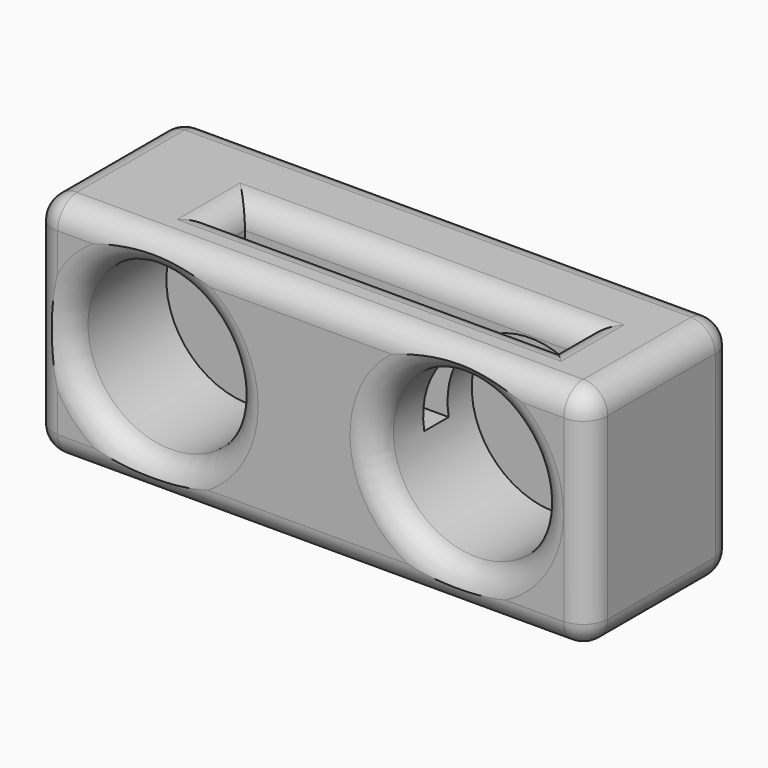
from build123d import *

# Parameters (mm, degrees)
F0_W          = 134.4953402877
F0_H          = 47.3678857088
F1_DEPTH      = 38.1
F2_R          = 17.202838431
F3_DEPTH      = 25.4
F4_W          = 69.85
F4_H          = 6.35
F5_DEPTH      = 25.4
F6_DEPTH      = 19.05
F7_T1_DEPTH   = 105.2834089168
F7_T3_DEPTH   = 27.9380686292
F7_T5_DEPTH   = 37.205954338
F7_T7_DEPTH   = 69.85
F7_T9_DEPTH   = 6.35
F7_S13_W      = 5.589502254
F7_S13_H      = 5.5895022539
F7_T14_DEPTH  = 5.589502254
F7_S19_W      = 5.5895022539
F7_S19_H      = 5.589502254
F7_T20_DEPTH  = 5.589502254
F7_S25_W      = 5.589502254
F7_S25_H      = 5.5895022539
F7_T26_DEPTH  = 5.589502254
F7_S31_W      = 5.5895022539
F7_S31_H      = 5.589502254
F7_T32_DEPTH  = 5.589502254
F7_S37_W      = 5.589502254
F7_S37_H      = 5.5895022539
F7_T38_DEPTH  = 5.589502254
F7_S43_W      = 5.5895022539
F7_S43_H      = 5.5895022539
F7_T44_DEPTH  = 5.589502254
F7_S49_W      = 5.589502254
F7_S49_H      = 5.5895022539
F7_T50_DEPTH  = 5.589502254
F7_S55_W      = 5.5895022539
F7_S55_H      = 5.5895022539
F7_T56_DEPTH  = 5.589502254
F7_T67_DEPTH  = 82.5524142529
F7_T71_DEPTH  = 19.0524142529
F7_T78_DEPTH  = 82.5524142529
F7_T82_DEPTH  = 19.0524142529
F7_T89_DEPTH  = 19.0524142529
F7_T93_DEPTH  = 82.5524142529
F7_T100_DEPTH = 19.0524142529
F7_T104_DEPTH = 82.5524142529


# Not quite as in the source:
# - a fillet or chamfer that OpenCascade refuses, or shapes differently, is made with other operations: its cross-section is extruded or revolved along the edge and cut away or added


with BuildPart() as f1:
    # F0 (on Front) → F1 (new body)
    with BuildSketch(Plane.XZ):
        with Locations((1.4725737274, 23.6839428544)):
            Rectangle(F0_W, F0_H)
    extrude(amount=F1_DEPTH)

    # F2 (on face) → F3 (cut)
    with BuildSketch(Plane.XZ.offset(38.1)):
        with Locations((-41.2180274725, 23.8331388682)):
            Circle(F2_R)
        with Locations((22.3340820521, 24.7883740813)):
            Circle(F2_R)
    extrude(amount=-F3_DEPTH, mode=Mode.SUBTRACT)

    # F4 (on face) → F5 (cut)
    with BuildSketch(Plane.XY.offset(47.3678857088)):
        with Locations((-2.1010648489, -22.1751800656)):
            Rectangle(F4_W, F4_H)
    extrude(amount=-F5_DEPTH, mode=Mode.SUBTRACT)

    # F6 (cut): a face of the model
    f6_faces = [f1.faces().sort_by_distance(p)[0] for p in [
        (68.7202438712, -19.05, 23.6839428544),
    ]]
    extrude(f6_faces, amount=-F6_DEPTH, mode=Mode.SUBTRACT)

    # F7: fillet of radius 5.08 on 18 edges, made by hand

    # F7_s2 → F7_t1 (cut)
    with BuildSketch(Plane.YZ.offset(-60.694130731)):
        with BuildLine():
            ThreePointArc((-33.0190343146, 47.3682857088), (-36.6121024484, 45.8799881572), (-38.1004, 42.2869200234))
            Line((-38.1004, 42.2869200234), (-38.6085365685, 42.2869200234))
            ThreePointArc((-38.6085365685, 42.2869200234), (-38.6081365685, 44.8274028661), (-38.6081365685, 47.3678857088))
            Line((-38.6081365685, 47.3678857088), (-38.1, 47.8760222774))
            ThreePointArc((-38.1, 47.8760222774), (-35.5595171573, 47.8760222774), (-33.0190343146, 47.8764222774))
            Line((-33.0190343146, 47.8764222774), (-33.0190343146, 47.3682857088))
        make_face()
        with BuildLine():
            ThreePointArc((-5.0809656854, 47.3682857088), (-1.4878975516, 45.8799881572), (0.0004, 42.2869200234))
            Line((0.0004, 42.2869200234), (0.5085365685, 42.2869200234))
            ThreePointArc((0.5085365685, 42.2869200234), (0.5081365685, 44.8274028661), (0.5081365685, 47.3678857088))
            Line((0.5081365685, 47.3678857088), (0, 47.8760222774))
            ThreePointArc((0, 47.8760222774), (-2.5404828427, 47.8760222774), (-5.0809656854, 47.8764222774))
            Line((-5.0809656854, 47.8764222774), (-5.0809656854, 47.3682857088))
        make_face()
        with BuildLine():
            ThreePointArc((-33.0190343146, -0.0004), (-36.6121024484, 1.4878975516), (-38.1004, 5.0809656854))
            Line((-38.1004, 5.0809656854), (-38.6085365685, 5.0809656854))
            ThreePointArc((-38.6085365685, 5.0809656854), (-38.6081365685, 2.5404828427), (-38.6081365685, 0))
            Line((-38.6081365685, 0), (-38.1, -0.5081365685))
            ThreePointArc((-38.1, -0.5081365685), (-35.5595171573, -0.5081365685), (-33.0190343146, -0.5085365685))
            Line((-33.0190343146, -0.5085365685), (-33.0190343146, -0.0004))
        make_face()
        with BuildLine():
            ThreePointArc((-5.0809656854, -0.0004), (-1.4878975516, 1.4878975516), (0.0004, 5.0809656854))
            Line((0.0004, 5.0809656854), (0.5085365685, 5.0809656854))
            ThreePointArc((0.5085365685, 5.0809656854), (0.5081365685, 2.5404828427), (0.5081365685, 0))
            Line((0.5081365685, 0), (0, -0.5081365685))
            ThreePointArc((0, -0.5081365685), (-2.5404828427, -0.5081365685), (-5.0809656854, -0.5085365685))
            Line((-5.0809656854, -0.5085365685), (-5.0809656854, -0.0004))
        make_face()
    extrude(amount=F7_T1_DEPTH, mode=Mode.SUBTRACT)

    # F7_s4 → F7_t3 (cut)
    with BuildSketch(Plane.XZ.offset(5.0809656854)):
        with BuildLine():
            ThreePointArc((44.5892781858, 47.3682857088), (48.1823463196, 45.8799881572), (49.6706438712, 42.2869200234))
            Line((49.6706438712, 42.2869200234), (50.1787804398, 42.2869200234))
            ThreePointArc((50.1787804398, 42.2869200234), (50.1783804398, 44.8274028661), (50.1783804398, 47.3678857088))
            Line((50.1783804398, 47.3678857088), (49.6702438712, 47.8760222774))
            ThreePointArc((49.6702438712, 47.8760222774), (47.1297610285, 47.8760222774), (44.5892781858, 47.8764222774))
            Line((44.5892781858, 47.8764222774), (44.5892781858, 47.3682857088))
        make_face()
        with BuildLine():
            ThreePointArc((-65.7754964165, 42.2869200234), (-64.2871988649, 45.8799881572), (-60.694130731, 47.3682857088))
            Line((-60.694130731, 47.3682857088), (-60.694130731, 47.8764222774))
            ThreePointArc((-60.694130731, 47.8764222774), (-63.2346135738, 47.8760222774), (-65.7750964165, 47.8760222774))
            Line((-65.7750964165, 47.8760222774), (-66.283232985, 47.3678857088))
            ThreePointArc((-66.283232985, 47.3678857088), (-66.283232985, 44.8274028661), (-66.283632985, 42.2869200234))
            Line((-66.283632985, 42.2869200234), (-65.7754964165, 42.2869200234))
        make_face()
        with BuildLine():
            ThreePointArc((44.5892781858, -0.0004), (48.1823463196, 1.4878975516), (49.6706438712, 5.0809656854))
            Line((49.6706438712, 5.0809656854), (50.1787804398, 5.0809656854))
            ThreePointArc((50.1787804398, 5.0809656854), (50.1783804398, 2.5404828427), (50.1783804398, 0))
            Line((50.1783804398, 0), (49.6702438712, -0.5081365685))
            ThreePointArc((49.6702438712, -0.5081365685), (47.1297610285, -0.5081365685), (44.5892781858, -0.5085365685))
            Line((44.5892781858, -0.5085365685), (44.5892781858, -0.0004))
        make_face()
        with BuildLine():
            ThreePointArc((-65.7754964165, 5.0809656854), (-64.2871988649, 1.4878975516), (-60.694130731, -0.0004))
            Line((-60.694130731, -0.0004), (-60.694130731, -0.5085365685))
            ThreePointArc((-60.694130731, -0.5085365685), (-63.2346135738, -0.5081365685), (-65.7750964165, -0.5081365685))
            Line((-65.7750964165, -0.5081365685), (-66.283232985, 0))
            ThreePointArc((-66.283232985, 0), (-66.283232985, 2.5404828427), (-66.283632985, 5.0809656854))
            Line((-66.283632985, 5.0809656854), (-65.7754964165, 5.0809656854))
        make_face()
    extrude(amount=F7_T3_DEPTH, mode=Mode.SUBTRACT)

    # F7_s6 → F7_t5 (cut)
    with BuildSketch(Plane.XY.offset(5.0809656854)):
        with BuildLine():
            ThreePointArc((44.5892781858, -38.1004), (48.1823463196, -36.6121024484), (49.6706438712, -33.0190343146))
            Line((49.6706438712, -33.0190343146), (50.1787804398, -33.0190343146))
            ThreePointArc((50.1787804398, -33.0190343146), (50.1783804398, -35.5595171573), (50.1783804398, -38.1))
            Line((50.1783804398, -38.1), (49.6702438712, -38.6081365685))
            ThreePointArc((49.6702438712, -38.6081365685), (47.1297610285, -38.6081365685), (44.5892781858, -38.6085365685))
            Line((44.5892781858, -38.6085365685), (44.5892781858, -38.1004))
        make_face()
        with BuildLine():
            ThreePointArc((-65.7754964165, -33.0190343146), (-64.2871988649, -36.6121024484), (-60.694130731, -38.1004))
            Line((-60.694130731, -38.1004), (-60.694130731, -38.6085365685))
            ThreePointArc((-60.694130731, -38.6085365685), (-63.2346135738, -38.6081365685), (-65.7750964165, -38.6081365685))
            Line((-65.7750964165, -38.6081365685), (-66.283232985, -38.1))
            ThreePointArc((-66.283232985, -38.1), (-66.283232985, -35.5595171573), (-66.283632985, -33.0190343146))
            Line((-66.283632985, -33.0190343146), (-65.7754964165, -33.0190343146))
        make_face()
        with BuildLine():
            ThreePointArc((44.5892781858, 0.0004), (48.1823463196, -1.4878975516), (49.6706438712, -5.0809656854))
            Line((49.6706438712, -5.0809656854), (50.1787804398, -5.0809656854))
            ThreePointArc((50.1787804398, -5.0809656854), (50.1783804398, -2.5404828427), (50.1783804398, 0))
            Line((50.1783804398, 0), (49.6702438712, 0.5081365685))
            ThreePointArc((49.6702438712, 0.5081365685), (47.1297610285, 0.5081365685), (44.5892781858, 0.5085365685))
            Line((44.5892781858, 0.5085365685), (44.5892781858, 0.0004))
        make_face()
        with BuildLine():
            ThreePointArc((-65.7754964165, -5.0809656854), (-64.2871988649, -1.4878975516), (-60.694130731, 0.0004))
            Line((-60.694130731, 0.0004), (-60.694130731, 0.5085365685))
            ThreePointArc((-60.694130731, 0.5085365685), (-63.2346135738, 0.5081365685), (-65.7750964165, 0.5081365685))
            Line((-65.7750964165, 0.5081365685), (-66.283232985, 0))
            ThreePointArc((-66.283232985, 0), (-66.283232985, -2.5404828427), (-66.283632985, -5.0809656854))
            Line((-66.283632985, -5.0809656854), (-65.7754964165, -5.0809656854))
        make_face()
    extrude(amount=F7_T5_DEPTH, mode=Mode.SUBTRACT)

    # F7_s8 → F7_t7 (cut)
    with BuildSketch(Plane.YZ.offset(-37.0260648489)):
        with BuildLine():
            ThreePointArc((-30.4311457511, 47.3682857088), (-26.8380776172, 45.8799881572), (-25.3497800656, 42.2869200234))
            Line((-25.3497800656, 42.2869200234), (-24.8416434971, 42.2869200234))
            ThreePointArc((-24.8416434971, 42.2869200234), (-24.8420434971, 44.8274028661), (-24.8420434971, 47.3678857088))
            Line((-24.8420434971, 47.3678857088), (-25.3501800656, 47.8760222774))
            ThreePointArc((-25.3501800656, 47.8760222774), (-27.8906629083, 47.8760222774), (-30.4311457511, 47.8764222774))
            Line((-30.4311457511, 47.8764222774), (-30.4311457511, 47.3682857088))
        make_face()
        with BuildLine():
            ThreePointArc((-13.9192143802, 47.3682857088), (-17.5122825141, 45.8799881572), (-19.0005800656, 42.2869200234))
            Line((-19.0005800656, 42.2869200234), (-19.5087166342, 42.2869200234))
            ThreePointArc((-19.5087166342, 42.2869200234), (-19.5083166342, 44.8274028661), (-19.5083166342, 47.3678857088))
            Line((-19.5083166342, 47.3678857088), (-19.0001800656, 47.8760222774))
            ThreePointArc((-19.0001800656, 47.8760222774), (-16.4596972229, 47.8760222774), (-13.9192143802, 47.8764222774))
            Line((-13.9192143802, 47.8764222774), (-13.9192143802, 47.3682857088))
        make_face()
    extrude(amount=F7_T7_DEPTH, mode=Mode.SUBTRACT)

    # F7_s10 → F7_t9 (cut)
    with BuildSketch(Plane.XZ.offset(19.0001800656)):
        with BuildLine():
            ThreePointArc((37.9049008365, 47.3682857088), (34.3118327027, 45.8799881572), (32.8235351511, 42.2869200234))
            Line((32.8235351511, 42.2869200234), (32.3153985826, 42.2869200234))
            ThreePointArc((32.3153985826, 42.2869200234), (32.3157985826, 44.8274028661), (32.3157985826, 47.3678857088))
            Line((32.3157985826, 47.3678857088), (32.8239351511, 47.8760222774))
            ThreePointArc((32.8239351511, 47.8760222774), (35.3644179938, 47.8760222774), (37.9049008365, 47.8764222774))
            Line((37.9049008365, 47.8764222774), (37.9049008365, 47.3682857088))
        make_face()
        with BuildLine():
            ThreePointArc((-42.1070305343, 47.3682857088), (-38.5139624005, 45.8799881572), (-37.0256648489, 42.2869200234))
            Line((-37.0256648489, 42.2869200234), (-36.5175282804, 42.2869200234))
            ThreePointArc((-36.5175282804, 42.2869200234), (-36.5179282804, 44.8274028661), (-36.5179282804, 47.3678857088))
            Line((-36.5179282804, 47.3678857088), (-37.0260648489, 47.8760222774))
            ThreePointArc((-37.0260648489, 47.8760222774), (-39.5665476916, 47.8760222774), (-42.1070305343, 47.8764222774))
            Line((-42.1070305343, 47.8764222774), (-42.1070305343, 47.3682857088))
        make_face()
    extrude(amount=F7_T9_DEPTH, mode=Mode.SUBTRACT)


with BuildPart() as f7_tool12:
    # F7_s13 → F7_t14 (new body)
    with BuildSketch(Plane.XY.offset(42.2869200234)):
        with Locations((47.3840293128, -35.8137854415)):
            Rectangle(F7_S13_W, F7_S13_H)
    extrude(amount=F7_T14_DEPTH)

    # F7_s15 → F7_t16 (revolve, cut)
    with BuildSketch(Plane(origin=(44.5892781858, -33.0190343146, 42.2869200234), x_dir=(-0.7071067812, 0.7071067812, 0), z_dir=(0.7071067812, 0.7071067812, 0))):
        with BuildLine():
            ThreePointArc((0, -5.0813656854), (5.0813656854, 0), (0, 5.0813656854))
            Line((0, 5.0813656854), (0, -5.0813656854))
        make_face()
    revolve(axis=Axis((44.5892781858, -33.0190343146, 42.2869200234), (0, 0, 1)), mode=Mode.SUBTRACT)


with BuildPart() as f1_1:
    add(f1.part)

    # F7_t11: cut F7_tool12
    add(f7_tool12.part, mode=Mode.SUBTRACT)


with BuildPart() as f7_tool18:
    # F7_s19 → F7_t20 (new body)
    with BuildSketch(Plane.YZ.offset(-60.694130731)):
        with Locations((-35.8137854415, 45.0816711504)):
            Rectangle(F7_S19_W, F7_S19_H)
    extrude(amount=-F7_T20_DEPTH)

    # F7_s21 → F7_t22 (revolve, cut)
    with BuildSketch(Plane(origin=(-60.694130731, -33.0190343146, 42.2869200234), x_dir=(0, 0.7071067812, -0.7071067812), z_dir=(0, 0.7071067812, 0.7071067812))):
        with BuildLine():
            ThreePointArc((0, -5.0813656854), (5.0813656854, 0), (0, 5.0813656854))
            Line((0, 5.0813656854), (0, -5.0813656854))
        make_face()
    revolve(axis=Axis((-60.694130731, -33.0190343146, 42.2869200234), (-1, 0, 0)), mode=Mode.SUBTRACT)


with BuildPart() as f1_2:
    add(f1_1.part)

    # F7_t17: cut F7_tool18
    add(f7_tool18.part, mode=Mode.SUBTRACT)


with BuildPart() as f7_tool24:
    # F7_s25 → F7_t26 (new body)
    with BuildSketch(Plane.XY.offset(42.2869200234)):
        with Locations((47.3840293128, -2.2862145584)):
            Rectangle(F7_S25_W, F7_S25_H)
    extrude(amount=F7_T26_DEPTH)

    # F7_s27 → F7_t28 (revolve, cut)
    with BuildSketch(Plane(origin=(44.5892781858, -5.0809656854, 42.2869200234), x_dir=(-0.7071067812, -0.7071067812, 0), z_dir=(-0.7071067812, 0.7071067812, 0))):
        with BuildLine():
            ThreePointArc((0, -5.0813656854), (5.0813656854, 0), (0, 5.0813656854))
            Line((0, 5.0813656854), (0, -5.0813656854))
        make_face()
    revolve(axis=Axis((44.5892781858, -5.0809656854, 42.2869200234), (0, 0, 1)), mode=Mode.SUBTRACT)


with BuildPart() as f1_3:
    add(f1_2.part)

    # F7_t23: cut F7_tool24
    add(f7_tool24.part, mode=Mode.SUBTRACT)


with BuildPart() as f7_tool30:
    # F7_s31 → F7_t32 (new body)
    with BuildSketch(Plane.YZ.offset(-60.694130731)):
        with Locations((-2.2862145584, 45.0816711504)):
            Rectangle(F7_S31_W, F7_S31_H)
    extrude(amount=-F7_T32_DEPTH)

    # F7_s33 → F7_t34 (revolve, cut)
    with BuildSketch(Plane(origin=(-60.694130731, -5.0809656854, 42.2869200234), x_dir=(0, -0.7071067812, -0.7071067812), z_dir=(0, 0.7071067812, -0.7071067812))):
        with BuildLine():
            ThreePointArc((0, -5.0813656854), (5.0813656854, 0), (0, 5.0813656854))
            Line((0, 5.0813656854), (0, -5.0813656854))
        make_face()
    revolve(axis=Axis((-60.694130731, -5.0809656854, 42.2869200234), (-1, 0, 0)), mode=Mode.SUBTRACT)


with BuildPart() as f1_4:
    add(f1_3.part)

    # F7_t29: cut F7_tool30
    add(f7_tool30.part, mode=Mode.SUBTRACT)


with BuildPart() as f7_tool36:
    # F7_s37 → F7_t38 (new body)
    with BuildSketch(Plane.XY.offset(5.0809656854)):
        with Locations((47.3840293128, -35.8137854415)):
            Rectangle(F7_S37_W, F7_S37_H)
    extrude(amount=-F7_T38_DEPTH)

    # F7_s39 → F7_t40 (revolve, cut)
    with BuildSketch(Plane(origin=(44.5892781858, -33.0190343146, 5.0809656854), x_dir=(-0.7071067812, 0.7071067812, 0), z_dir=(-0.7071067812, -0.7071067812, 0))):
        with BuildLine():
            ThreePointArc((0, -5.0813656854), (5.0813656854, 0), (0, 5.0813656854))
            Line((0, 5.0813656854), (0, -5.0813656854))
        make_face()
    revolve(axis=Axis((44.5892781858, -33.0190343146, 5.0809656854), (0, 0, -1)), mode=Mode.SUBTRACT)


with BuildPart() as f1_5:
    add(f1_4.part)

    # F7_t35: cut F7_tool36
    add(f7_tool36.part, mode=Mode.SUBTRACT)


with BuildPart() as f7_tool42:
    # F7_s43 → F7_t44 (new body)
    with BuildSketch(Plane.YZ.offset(-60.694130731)):
        with Locations((-35.8137854415, 2.2862145584)):
            Rectangle(F7_S43_W, F7_S43_H)
    extrude(amount=-F7_T44_DEPTH)

    # F7_s45 → F7_t46 (revolve, cut)
    with BuildSketch(Plane(origin=(-60.694130731, -33.0190343146, 5.0809656854), x_dir=(0, 0.7071067812, 0.7071067812), z_dir=(0, -0.7071067812, 0.7071067812))):
        with BuildLine():
            ThreePointArc((0, -5.0813656854), (5.0813656854, 0), (0, 5.0813656854))
            Line((0, 5.0813656854), (0, -5.0813656854))
        make_face()
    revolve(axis=Axis((-60.694130731, -33.0190343146, 5.0809656854), (-1, 0, 0)), mode=Mode.SUBTRACT)


with BuildPart() as f1_6:
    add(f1_5.part)

    # F7_t41: cut F7_tool42
    add(f7_tool42.part, mode=Mode.SUBTRACT)


with BuildPart() as f7_tool48:
    # F7_s49 → F7_t50 (new body)
    with BuildSketch(Plane.XY.offset(5.0809656854)):
        with Locations((47.3840293128, -2.2862145584)):
            Rectangle(F7_S49_W, F7_S49_H)
    extrude(amount=-F7_T50_DEPTH)

    # F7_s51 → F7_t52 (revolve, cut)
    with BuildSketch(Plane(origin=(44.5892781858, -5.0809656854, 5.0809656854), x_dir=(-0.7071067812, -0.7071067812, 0), z_dir=(0.7071067812, -0.7071067812, 0))):
        with BuildLine():
            ThreePointArc((0, -5.0813656854), (5.0813656854, 0), (0, 5.0813656854))
            Line((0, 5.0813656854), (0, -5.0813656854))
        make_face()
    revolve(axis=Axis((44.5892781858, -5.0809656854, 5.0809656854), (0, 0, -1)), mode=Mode.SUBTRACT)


with BuildPart() as f1_7:
    add(f1_6.part)

    # F7_t47: cut F7_tool48
    add(f7_tool48.part, mode=Mode.SUBTRACT)


with BuildPart() as f7_tool54:
    # F7_s55 → F7_t56 (new body)
    with BuildSketch(Plane.YZ.offset(-60.694130731)):
        with Locations((-2.2862145584, 2.2862145584)):
            Rectangle(F7_S55_W, F7_S55_H)
    extrude(amount=-F7_T56_DEPTH)

    # F7_s57 → F7_t58 (revolve, cut)
    with BuildSketch(Plane(origin=(-60.694130731, -5.0809656854, 5.0809656854), x_dir=(0, -0.7071067812, 0.7071067812), z_dir=(0, -0.7071067812, -0.7071067812))):
        with BuildLine():
            ThreePointArc((0, -5.0813656854), (5.0813656854, 0), (0, 5.0813656854))
            Line((0, 5.0813656854), (0, -5.0813656854))
        make_face()
    revolve(axis=Axis((-60.694130731, -5.0809656854, 5.0809656854), (-1, 0, 0)), mode=Mode.SUBTRACT)


with BuildPart() as f1_8:
    add(f1_7.part)

    # F7_t53: cut F7_tool54
    add(f7_tool54.part, mode=Mode.SUBTRACT)

    # F7_s59 → F7_t60 (revolve, cut)
    with BuildSketch(Plane.XY.offset(23.8331388682)):
        with BuildLine():
            ThreePointArc((-18.9342233561, -38.1004), (-22.52729149, -36.6121024484), (-24.0155890415, -33.0190343146))
            Line((-24.0155890415, -33.0190343146), (-24.5237256101, -33.0190343146))
            ThreePointArc((-24.5237256101, -33.0190343146), (-24.5233256101, -35.5595171573), (-24.5233256101, -38.1))
            Line((-24.5233256101, -38.1), (-24.0151890415, -38.6081365685))
            ThreePointArc((-24.0151890415, -38.6081365685), (-21.4747061988, -38.6081365685), (-18.9342233561, -38.6085365685))
            Line((-18.9342233561, -38.6085365685), (-18.9342233561, -38.1004))
        make_face()
    revolve(axis=Axis((-41.2180274725, -38.1, 23.8331388682), (0, -1, 0)), mode=Mode.SUBTRACT)

    # F7_s61 → F7_t62 (revolve, cut)
    with BuildSketch(Plane.XY.offset(24.7883740813)):
        with BuildLine():
            ThreePointArc((44.6178861685, -38.1004), (41.0248180346, -36.6121024484), (39.5365204831, -33.0190343146))
            Line((39.5365204831, -33.0190343146), (39.0283839145, -33.0190343146))
            ThreePointArc((39.0283839145, -33.0190343146), (39.0287839145, -35.5595171573), (39.0287839145, -38.1))
            Line((39.0287839145, -38.1), (39.5369204831, -38.6081365685))
            ThreePointArc((39.5369204831, -38.6081365685), (42.0774033258, -38.6081365685), (44.6178861685, -38.6085365685))
            Line((44.6178861685, -38.6085365685), (44.6178861685, -38.1004))
        make_face()
    revolve(axis=Axis((22.3340820521, -38.1, 24.7883740813), (0, -1, 0)), mode=Mode.SUBTRACT)


with BuildPart() as f7_tool65:
    # F7_s66 → F7_t67 (new body)
    with BuildSketch(Plane.YZ.offset(-49.7284791018)):
        with BuildLine():
            ThreePointArc((-30.4311457511, 47.3682857088), (-26.8380776172, 45.8799881572), (-25.3497800656, 42.2869200234))
            Line((-25.3497800656, 42.2869200234), (-24.8416434971, 42.2869200234))
            ThreePointArc((-24.8416434971, 42.2869200234), (-24.8420434971, 44.8274028661), (-24.8420434971, 47.3678857088))
            Line((-24.8420434971, 47.3678857088), (-25.3501800656, 47.8760222774))
            ThreePointArc((-25.3501800656, 47.8760222774), (-27.8906629083, 47.8760222774), (-30.4311457511, 47.8764222774))
            Line((-30.4311457511, 47.8764222774), (-30.4311457511, 47.3682857088))
        make_face()
    extrude(amount=F7_T67_DEPTH)

    split(bisect_by=Plane.YZ.offset(-37.0260648489), keep=Keep.BOTTOM)


with BuildPart() as f7_tool69:
    # F7_s70 → F7_t71 (new body)
    with BuildSketch(Plane.XZ.offset(19.0001800656)):
        with BuildLine():
            ThreePointArc((-42.1070305343, 47.3682857088), (-38.5139624005, 45.8799881572), (-37.0256648489, 42.2869200234))
            Line((-37.0256648489, 42.2869200234), (-36.5175282804, 42.2869200234))
            ThreePointArc((-36.5175282804, 42.2869200234), (-36.5179282804, 44.8274028661), (-36.5179282804, 47.3678857088))
            Line((-36.5179282804, 47.3678857088), (-37.0260648489, 47.8760222774))
            ThreePointArc((-37.0260648489, 47.8760222774), (-39.5665476916, 47.8760222774), (-42.1070305343, 47.8764222774))
            Line((-42.1070305343, 47.8764222774), (-42.1070305343, 47.3682857088))
        make_face()
    extrude(amount=F7_T71_DEPTH)

    split(bisect_by=Plane.XZ.offset(25.3501800656), keep=Keep.TOP)


with BuildPart() as f7_tool65_1:
    add(f7_tool65.part)

    # F7_t73: intersect F7_tool69
    add(f7_tool69.part, mode=Mode.INTERSECT)


with BuildPart() as f1_9:
    add(f1_8.part)

    # F7_t63: cut F7_tool65
    add(f7_tool65_1.part, mode=Mode.SUBTRACT)


with BuildPart() as f7_tool76:
    # F7_s77 → F7_t78 (new body)
    with BuildSketch(Plane.YZ.offset(-37.0260648489)):
        with BuildLine():
            ThreePointArc((-30.4311457511, 47.3682857088), (-26.8380776172, 45.8799881572), (-25.3497800656, 42.2869200234))
            Line((-25.3497800656, 42.2869200234), (-24.8416434971, 42.2869200234))
            ThreePointArc((-24.8416434971, 42.2869200234), (-24.8420434971, 44.8274028661), (-24.8420434971, 47.3678857088))
            Line((-24.8420434971, 47.3678857088), (-25.3501800656, 47.8760222774))
            ThreePointArc((-25.3501800656, 47.8760222774), (-27.8906629083, 47.8760222774), (-30.4311457511, 47.8764222774))
            Line((-30.4311457511, 47.8764222774), (-30.4311457511, 47.3682857088))
        make_face()
    extrude(amount=F7_T78_DEPTH)

    split(bisect_by=Plane.YZ.offset(32.8239351511), keep=Keep.TOP)


with BuildPart() as f7_tool80:
    # F7_s81 → F7_t82 (new body)
    with BuildSketch(Plane.XZ.offset(38.0525943186)):
        with BuildLine():
            ThreePointArc((37.9049008365, 47.3682857088), (34.3118327027, 45.8799881572), (32.8235351511, 42.2869200234))
            Line((32.8235351511, 42.2869200234), (32.3153985826, 42.2869200234))
            ThreePointArc((32.3153985826, 42.2869200234), (32.3157985826, 44.8274028661), (32.3157985826, 47.3678857088))
            Line((32.3157985826, 47.3678857088), (32.8239351511, 47.8760222774))
            ThreePointArc((32.8239351511, 47.8760222774), (35.3644179938, 47.8760222774), (37.9049008365, 47.8764222774))
            Line((37.9049008365, 47.8764222774), (37.9049008365, 47.3682857088))
        make_face()
    extrude(amount=-F7_T82_DEPTH)

    split(bisect_by=Plane.XZ.offset(25.3501800656), keep=Keep.TOP)


with BuildPart() as f7_tool76_1:
    add(f7_tool76.part)

    # F7_t84: intersect F7_tool80
    add(f7_tool80.part, mode=Mode.INTERSECT)


with BuildPart() as f1_10:
    add(f1_9.part)

    # F7_t74: cut F7_tool76
    add(f7_tool76_1.part, mode=Mode.SUBTRACT)


with BuildPart() as f7_tool87:
    # F7_s88 → F7_t89 (new body)
    with BuildSketch(Plane.XZ.offset(25.3501800656)):
        with BuildLine():
            ThreePointArc((37.9049008365, 47.3682857088), (34.3118327027, 45.8799881572), (32.8235351511, 42.2869200234))
            Line((32.8235351511, 42.2869200234), (32.3153985826, 42.2869200234))
            ThreePointArc((32.3153985826, 42.2869200234), (32.3157985826, 44.8274028661), (32.3157985826, 47.3678857088))
            Line((32.3157985826, 47.3678857088), (32.8239351511, 47.8760222774))
            ThreePointArc((32.8239351511, 47.8760222774), (35.3644179938, 47.8760222774), (37.9049008365, 47.8764222774))
            Line((37.9049008365, 47.8764222774), (37.9049008365, 47.3682857088))
        make_face()
    extrude(amount=-F7_T89_DEPTH)

    split(bisect_by=Plane.XZ.offset(19.0001800656), keep=Keep.BOTTOM)


with BuildPart() as f7_tool91:
    # F7_s92 → F7_t93 (new body)
    with BuildSketch(Plane.YZ.offset(45.526349404)):
        with BuildLine():
            ThreePointArc((-13.9192143802, 47.3682857088), (-17.5122825141, 45.8799881572), (-19.0005800656, 42.2869200234))
            Line((-19.0005800656, 42.2869200234), (-19.5087166342, 42.2869200234))
            ThreePointArc((-19.5087166342, 42.2869200234), (-19.5083166342, 44.8274028661), (-19.5083166342, 47.3678857088))
            Line((-19.5083166342, 47.3678857088), (-19.0001800656, 47.8760222774))
            ThreePointArc((-19.0001800656, 47.8760222774), (-16.4596972229, 47.8760222774), (-13.9192143802, 47.8764222774))
            Line((-13.9192143802, 47.8764222774), (-13.9192143802, 47.3682857088))
        make_face()
    extrude(amount=-F7_T93_DEPTH)

    split(bisect_by=Plane.YZ.offset(32.8239351511), keep=Keep.TOP)


with BuildPart() as f7_tool87_1:
    add(f7_tool87.part)

    # F7_t95: intersect F7_tool91
    add(f7_tool91.part, mode=Mode.INTERSECT)


with BuildPart() as f1_11:
    add(f1_10.part)

    # F7_t85: cut F7_tool87
    add(f7_tool87_1.part, mode=Mode.SUBTRACT)


with BuildPart() as f7_tool98:
    # F7_s99 → F7_t100 (new body)
    with BuildSketch(Plane.XZ.offset(6.2977658127)):
        with BuildLine():
            ThreePointArc((-42.1070305343, 47.3682857088), (-38.5139624005, 45.8799881572), (-37.0256648489, 42.2869200234))
            Line((-37.0256648489, 42.2869200234), (-36.5175282804, 42.2869200234))
            ThreePointArc((-36.5175282804, 42.2869200234), (-36.5179282804, 44.8274028661), (-36.5179282804, 47.3678857088))
            Line((-36.5179282804, 47.3678857088), (-37.0260648489, 47.8760222774))
            ThreePointArc((-37.0260648489, 47.8760222774), (-39.5665476916, 47.8760222774), (-42.1070305343, 47.8764222774))
            Line((-42.1070305343, 47.8764222774), (-42.1070305343, 47.3682857088))
        make_face()
    extrude(amount=F7_T100_DEPTH)

    split(bisect_by=Plane.XZ.offset(19.0001800656), keep=Keep.BOTTOM)


with BuildPart() as f7_tool102:
    # F7_s103 → F7_t104 (new body)
    with BuildSketch(Plane.YZ.offset(32.8239351511)):
        with BuildLine():
            ThreePointArc((-13.9192143802, 47.3682857088), (-17.5122825141, 45.8799881572), (-19.0005800656, 42.2869200234))
            Line((-19.0005800656, 42.2869200234), (-19.5087166342, 42.2869200234))
            ThreePointArc((-19.5087166342, 42.2869200234), (-19.5083166342, 44.8274028661), (-19.5083166342, 47.3678857088))
            Line((-19.5083166342, 47.3678857088), (-19.0001800656, 47.8760222774))
            ThreePointArc((-19.0001800656, 47.8760222774), (-16.4596972229, 47.8760222774), (-13.9192143802, 47.8764222774))
            Line((-13.9192143802, 47.8764222774), (-13.9192143802, 47.3682857088))
        make_face()
    extrude(amount=-F7_T104_DEPTH)

    split(bisect_by=Plane.YZ.offset(-37.0260648489), keep=Keep.BOTTOM)


with BuildPart() as f7_tool98_1:
    add(f7_tool98.part)

    # F7_t106: intersect F7_tool102
    add(f7_tool102.part, mode=Mode.INTERSECT)


with BuildPart() as f1_12:
    add(f1_11.part)

    # F7_t96: cut F7_tool98
    add(f7_tool98_1.part, mode=Mode.SUBTRACT)


solid = f1_12.part
